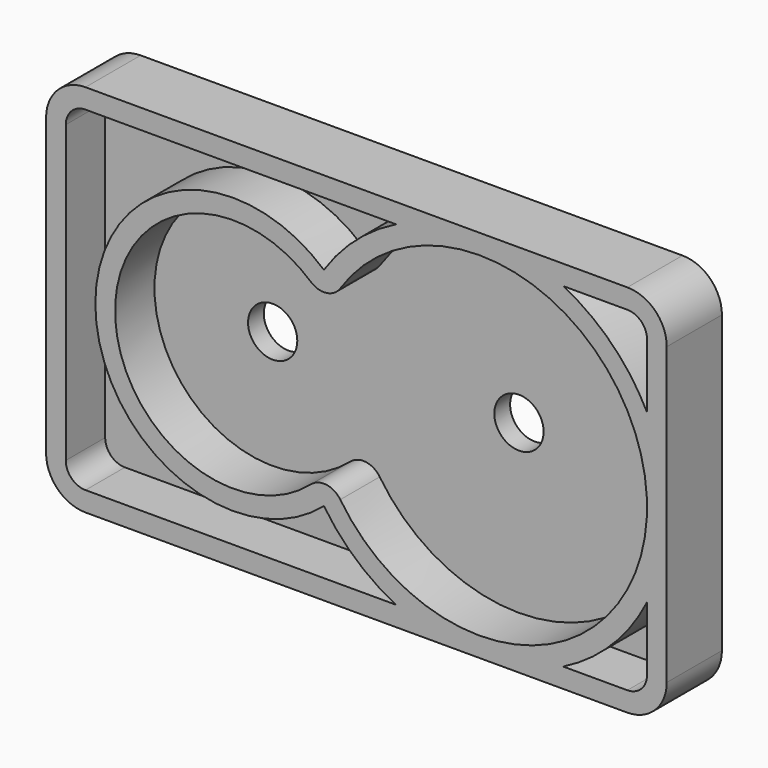
from build123d import *

# Parameters (mm, degrees)
F1_DEPTH     = 5
F3_DEPTH     = 2
F4_T         = 2
F4_T4_ANGLE  = 97.3436104927
F4_T6_ANGLE  = 292.5225547035
F4_T8_ANGLE  = 97.3436104927
F4_T10_ANGLE = 262.1646662819
F5_R         = 2.5
F6_DEPTH     = 2


# Not quite as in the source:
# - a shell that OpenCascade refuses in one call is made with other operations: the cavity is built on its own and cut out


with BuildPart() as f1:
    # F0 (on Front) → F1 (new body)
    with BuildSketch(Plane.XZ):
        with BuildLine():
            ThreePointArc((31.5, 15), (30.3284271247, 17.8284271247), (27.5, 19))
            Line((27.5, 19), (-27.5, 19))
            ThreePointArc((-27.5, 19), (-30.3284271247, 17.8284271247), (-31.5, 15))
            Line((-31.5, 15), (-31.5, -15))
            ThreePointArc((-31.5, -15), (-30.3284271247, -17.8284271247), (-27.5, -19))
            Line((-27.5, -19), (27.5, -19))
            ThreePointArc((27.5, -19), (30.3284271247, -17.8284271247), (31.5, -15))
            Line((31.5, -15), (31.5, 15))
        make_face()
        with BuildLine():
            ThreePointArc((-1.6368421053, 9.4419116333), (29.5, 0), (-1.6368421053, -9.4419116333))
            ThreePointArc((-1.6368421053, -9.4419116333), (-3.0358514886, -8.5702451163), (-4.6142857143, -9.0451926571))
            ThreePointArc((-4.6142857143, -9.0451926571), (-24.5, 0), (-4.6142857143, 9.0451926571))
            ThreePointArc((-4.6142857143, 9.0451926571), (-3.0358514886, 8.5702451163), (-1.6368421053, 9.4419116333))
        make_face(mode=Mode.SUBTRACT)
    extrude(amount=F1_DEPTH)

    # F2 (on face) → F3 (join)
    with BuildSketch(Plane(origin=(0, 0, 0), x_dir=(-1, 0, 0), z_dir=(0, 1, 0))):
        with BuildLine():
            Line((27.5, 19), (-27.5, 19))
            ThreePointArc((-27.5, 19), (-30.3284271247, 17.8284271247), (-31.5, 15))
            Line((-31.5, 15), (-31.5, -15))
            ThreePointArc((-31.5, -15), (-30.3284271247, -17.8284271247), (-27.5, -19))
            Line((-27.5, -19), (27.5, -19))
            ThreePointArc((27.5, -19), (30.3284271247, -17.8284271247), (31.5, -15))
            Line((31.5, -15), (31.5, 15))
            ThreePointArc((31.5, 15), (30.3284271247, 17.8284271247), (27.5, 19))
        make_face()
    extrude(amount=F3_DEPTH)

    # F4: shell of thickness 2, made by hand


with BuildPart() as f4_core1:
    # F4_t2: copy of F1
    add(f1.part)

    # the walls: a layer under each face that stays
    f4_faces = [f4_core1.faces().sort_by_distance(p)[0] for p in [
        (30.3284271247, -1.5, 17.8284271247),
        (0, 2, 0),
        (-30.3284271247, -1.5, 17.8284271247),
        (-31.5, -1.5, 0),
        (-30.3284271247, -1.5, -17.8284271247),
        (0, -1.5, -19),
        (30.3284271247, -1.5, -17.8284271247),
        (0, -1.5, 19),
        (2.5, 0, 0),
        (29.5, -2.5, 0),
        (-24.5, -2.5, 0),
        (31.5, -1.5, 0),
    ]]
    thicken(f4_faces, amount=-F4_T, mode=Mode.SUBTRACT)

    # F4_s3 → F4_t4 (revolve, cut)
    with BuildSketch(Plane(origin=(3.8559556787, 0, -5.7733051009), x_dir=(0, 1, 0), z_dir=(0.5554065667, 0, -0.8315789474))):
        Polygon((-0.02, -6.5852631579), (0, -8.6052631579), (2, -8.6052631579), (2, -6.6052631579), align=None)
    revolve(axis=Axis((-3.3, 0, -10.5527247666), (0, -1, 0)), revolution_arc=F4_T4_ANGLE, mode=Mode.SUBTRACT)

    # F4_s5 → F4_t6 (revolve, cut)
    with BuildSketch(Plane(origin=(3.8559556787, 0, 5.7733051009), x_dir=(0, 1, 0), z_dir=(-0.5554065667, 0, -0.8315789474))):
        Polygon((-0.02, -6.5852631579), (2, -6.6052631579), (2, -8.6052631579), (0, -8.6052631579), align=None)
    revolve(axis=Axis((12.5, 0, 0), (0, 1, 0)), revolution_arc=F4_T6_ANGLE, mode=Mode.SUBTRACT)

    # F4_s7 → F4_t8 (revolve, cut)
    with BuildSketch(Plane(origin=(-7.1020408163, 0, 6.1916497355), x_dir=(0, 1, 0), z_dir=(-0.7537660548, 0, 0.6571428571))):
        Polygon((-0.02, -3.7657142857), (2, -3.7857142857), (2, -5.7857142857), (0, -5.7857142857), align=None)
    revolve(axis=Axis((-3.3, 0, 10.5527247666), (0, -1, 0)), revolution_arc=F4_T8_ANGLE, mode=Mode.SUBTRACT)

    # F4_s9 → F4_t10 (revolve, cut)
    with BuildSketch(Plane(origin=(-7.1020408163, 0, -6.1916497355), x_dir=(0, 1, 0), z_dir=(0.7537660548, 0, 0.6571428571))):
        Polygon((-0.02, -3.7657142857), (2, -3.7857142857), (2, -5.7857142857), (0, -5.7857142857), align=None)
    revolve(axis=Axis((-12.5, 0, 0), (0, 1, 0)), revolution_arc=F4_T10_ANGLE, mode=Mode.SUBTRACT)


with BuildPart() as f1_1:
    add(f1.part)

    # what is left inside the walls is the cavity
    f4_cavity = [f4_core1.part.solids().sort_by_distance(p)[0] for p in [
        (25.949171, -3.333333, 13.449171),
        (25.949171, -3.333333, -13.449171),
        (-21.12132, -0.02, -13.222222),
    ]]
    add(f4_cavity, mode=Mode.SUBTRACT)

    # F5 (on face) → F6 (cut, through all)
    with BuildSketch(Plane.XZ):
        with Locations((-12.5, 0)):
            Circle(F5_R)
        with Locations((12.5, 0)):
            Circle(F5_R)
    extrude(amount=-F6_DEPTH, mode=Mode.SUBTRACT)


solid = f1_1.part
